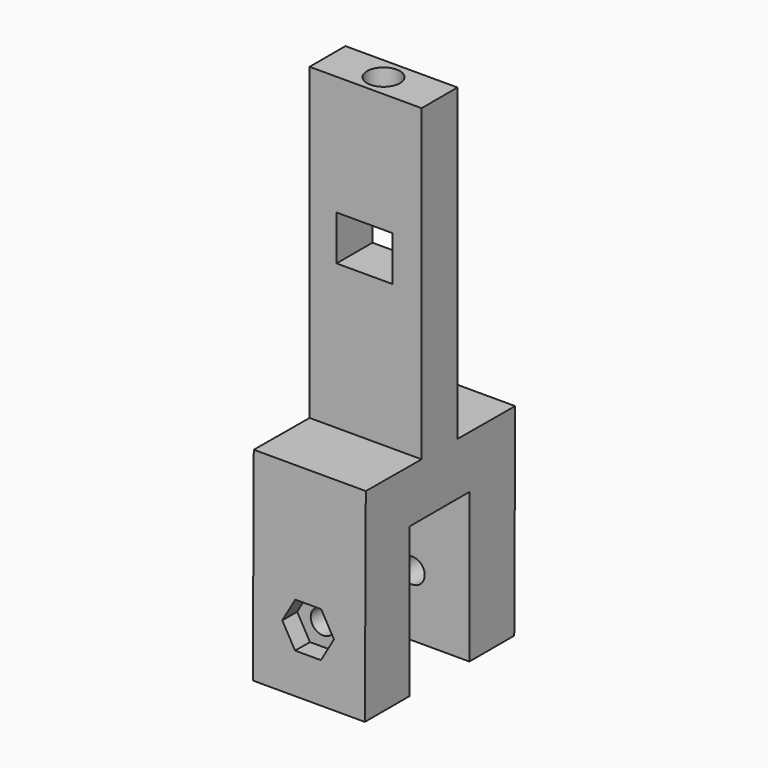
from build123d import *

# Parameters (mm, degrees)
F0_W     = 15
F0_H     = 43.4799888134
F0_W_2   = 7.5
F0_H_2   = 6
F1_DEPTH = 6
F3_DEPTH = 15
F5_D     = 4.4
F5_DEPTH = 20
F5_TIP   = 1.3218933619
F7_D     = 3.3
F7_DEPTH = 40
F7_TIP   = 0.9914200214
F8_DEPTH = 2.5


with BuildPart() as f1:
    # F0 (on Front) → F1 (new body)
    with BuildSketch(Plane.XZ):
        with Locations((0.1361690943, 49.7399944067)):
            Rectangle(F0_W, F0_H)
        with Locations((0, 52.4799888134)):
            Rectangle(F0_W_2, F0_H_2, mode=Mode.SUBTRACT)
    extrude(amount=F1_DEPTH)

    # F2 (on face) → F3 (join)
    with BuildSketch(Plane.YZ.offset(7.6361690943)):
        Polygon((9.5002116757, 3), (9.6573423812, 30), (0, 30.0562024082), (0, 28), (-6, 28), (-6, 30.0911203428), (-15.3422342746, 30.1454889303), (-15.5002116757, 3), (-8, 3), (-8, 23), (2, 23), (2, 3), align=None)
    extrude(amount=-F3_DEPTH)

    # F5
    with Locations(Plane.XY.offset(71.4799888134)):
        with Locations((0.1361690943, -3)):
            Hole(F5_D / 2, depth=F5_DEPTH)
            with Locations((0, 0, -(F5_DEPTH + F5_TIP / 2))):  # 118° drill point
                Cone(0, F5_D / 2, F5_TIP, mode=Mode.SUBTRACT)

    # F7
    with Locations(Plane(origin=(0, -15.5171451022, 0.0903044429), x_dir=(1, 0, 0), z_dir=(0, -0.9999830662, 0.0058195572))):
        with Locations((0, 11.2554198566)):
            Hole(F7_D / 2, depth=F7_DEPTH)
            with Locations((0, 0, -(F7_DEPTH + F7_TIP / 2))):  # 118° drill point
                Cone(0, F7_D / 2, F7_TIP, mode=Mode.SUBTRACT)

    # F6 (on face) → F8 (cut)
    with BuildSketch(Plane(origin=(0, -15.5171451022, 0.0903044429), x_dir=(1, 0, 0), z_dir=(0, -0.9999830662, 0.0058195572))):
        Polygon((1.7320508076, 14.2554198566), (-1.7320508076, 14.2554198566), (-3.4641016151, 11.2554198566), (-1.7320508076, 8.2554198566), (1.7320508076, 8.2554198566), (3.4641016151, 11.2554198566), align=None)
    extrude(amount=-F8_DEPTH, mode=Mode.SUBTRACT)


solid = f1.part
